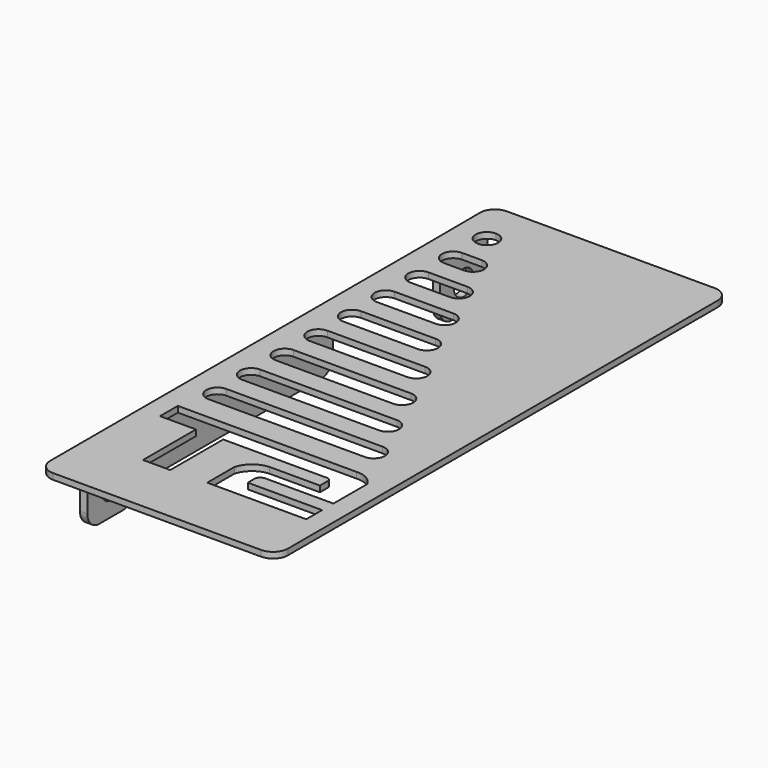
from build123d import *

# Parameters (mm, degrees)
F1_DEPTH = 1.2
F2_DEPTH = 15
F4_D     = 5
F5_R     = 3
F6_DEPTH = 3
F7_DEPTH = 12
F8_R     = 3


# Not quite as in the source:
# - a feature names something its author has since deleted; it is built from what else it names


with BuildPart() as f1:
    # F0 (on Top) → F1 (new body)
    with BuildSketch(Plane.XY):
        Polygon((24, 57.25), (-24, 57.25), (-24.0091441598, 54.25), (-22.5091511277, 54.2454279414), (-22.5091511277, 42.2454279414), (-22.5059426621, 15.2501562063), (-22.5, -34.75), (-22.5, -46.75), (-24, -46.75), (-24, -57.25), (24, -57.25), align=None)
        with BuildLine():
            Line((13.9209458456, -22.2416133583), (-17.6390541544, -22.2416133583))
            ThreePointArc((-17.6390541544, -22.2416133583), (-19.8890541544, -19.9916133583), (-17.6390541544, -17.7416133583))
            Line((-17.6390541544, -17.7416133583), (13.9209458456, -17.7416133583))
            ThreePointArc((13.9209458456, -17.7416133583), (16.1709458456, -19.9916133583), (13.9209458456, -22.2416133583))
        make_face(mode=Mode.SUBTRACT)
        with BuildLine():
            Line((9.9809458456, -13.7416133583), (-17.6390541544, -13.7416133583))
            ThreePointArc((-17.6390541544, -13.7416133583), (-19.8890541544, -11.4916133583), (-17.6390541544, -9.2416133583))
            Line((-17.6390541544, -9.2416133583), (9.9809458456, -9.2416133583))
            ThreePointArc((9.9809458456, -9.2416133583), (12.2309458456, -11.4916133583), (9.9809458456, -13.7416133583))
        make_face(mode=Mode.SUBTRACT)
        with BuildLine():
            Line((6.0409458456, -5.2416133583), (-17.6390541544, -5.2416133583))
            ThreePointArc((-17.6390541544, -5.2416133583), (-19.8890541544, -2.9916133583), (-17.6390541544, -0.7416133583))
            Line((-17.6390541544, -0.7416133583), (6.0409458456, -0.7416133583))
            ThreePointArc((6.0409458456, -0.7416133583), (8.2909458456, -2.9916133583), (6.0409458456, -5.2416133583))
        make_face(mode=Mode.SUBTRACT)
        with BuildLine():
            Line((-19.9999999992, -31.5317022603), (-19.9999999992, -27.0317022603))
            Line((-19.9999999992, -27.0317022603), (16.0951670268, -27.0317022603))
            ThreePointArc((16.0951670268, -27.0317022603), (18.3824934665, -27.555243649), (19.9999999704, -29.25513498))
            Line((19.9999999704, -29.25513498), (19.991580365, -37.75513498))
            Line((19.991580365, -37.75513498), (6.1573753969, -37.7551350426))
            ThreePointArc((6.1573753969, -37.7551350426), (5.4441089744, -38.037790108), (4.9890264818, -38.6554816172))
            Line((4.9890264818, -38.6554816172), (4.9890264818, -40.6197120801))
            Line((4.9890264818, -40.6197120801), (19.9890264818, -40.6197120801))
            Line((19.9890264818, -40.6197120801), (20, -44.6197120801))
            Line((20, -44.6197120801), (0, -44.6197120801))
            Line((0, -44.6197120801), (0, -37.7900532508))
            ThreePointArc((0, -37.7900532508), (1.5958871284, -35.3350022858), (4.3312619815, -34.2900834468))
            Line((4.3312619815, -34.2900834468), (14.5000001306, -34.2900834468))
            Line((14.5000001306, -34.2900834468), (14.5000000048, -32.3122422563))
            ThreePointArc((14.5000000048, -32.3122422563), (14.2713851276, -31.7603171319), (13.7194600008, -31.5317022603))
            Line((13.7194600008, -31.5317022603), (-7.2499999992, -31.5317022603))
            Line((-7.2499999992, -31.5317022603), (-7.2499999992, -44.8960133593))
            Line((-7.2499999992, -44.8960133593), (-12.7499999992, -44.8960133593))
            Line((-12.7499999992, -44.8960133593), (-12.7499999992, -31.5317022603))
            Line((-12.7499999992, -31.5317022603), (-19.9999999992, -31.5317022603))
        make_face(mode=Mode.SUBTRACT)
        with BuildLine():
            Line((2.1009458456, 3.2583866417), (-17.6390541544, 3.2583866417))
            ThreePointArc((-17.6390541544, 3.2583866417), (-19.8890541544, 5.5083866417), (-17.6390541544, 7.7583866417))
            Line((-17.6390541544, 7.7583866417), (2.1009458456, 7.7583866417))
            ThreePointArc((2.1009458456, 7.7583866417), (4.3509458456, 5.5083866417), (2.1009458456, 3.2583866417))
        make_face(mode=Mode.SUBTRACT)
        with BuildLine():
            Line((-2.5590541544, 11.7583866417), (-17.6390541544, 11.7583866417))
            ThreePointArc((-17.6390541544, 11.7583866417), (-19.8890541544, 14.0083866417), (-17.6390541544, 16.2583866417))
            Line((-17.6390541544, 16.2583866417), (-2.5590541544, 16.2583866417))
            ThreePointArc((-2.5590541544, 16.2583866417), (-0.3090541544, 14.0083866417), (-2.5590541544, 11.7583866417))
        make_face(mode=Mode.SUBTRACT)
        with BuildLine():
            Line((-5.7790541544, 20.2583866417), (-17.6390541544, 20.2583866417))
            ThreePointArc((-17.6390541544, 20.2583866417), (-19.8890541544, 22.5083866417), (-17.6390541544, 24.7583866417))
            Line((-17.6390541544, 24.7583866417), (-5.7790541544, 24.7583866417))
            ThreePointArc((-5.7790541544, 24.7583866417), (-3.5290541544, 22.5083866417), (-5.7790541544, 20.2583866417))
        make_face(mode=Mode.SUBTRACT)
        with BuildLine():
            Line((-9.7190541544, 28.7583866417), (-17.6390541544, 28.7583866417))
            ThreePointArc((-17.6390541544, 28.7583866417), (-19.8890541544, 31.0083866417), (-17.6390541544, 33.2583866417))
            Line((-17.6390541544, 33.2583866417), (-9.7190541544, 33.2583866417))
            ThreePointArc((-9.7190541544, 33.2583866417), (-7.4690541544, 31.0083866417), (-9.7190541544, 28.7583866417))
        make_face(mode=Mode.SUBTRACT)
        with BuildLine():
            Line((-13.6590541544, 37.2583866417), (-17.6390541544, 37.2583866417))
            ThreePointArc((-17.6390541544, 37.2583866417), (-19.8890541544, 39.5083866417), (-17.6390541544, 41.7583866417))
            Line((-17.6390541544, 41.7583866417), (-13.6590541544, 41.7583866417))
            ThreePointArc((-13.6590541544, 41.7583866417), (-11.4090541544, 39.5083866417), (-13.6590541544, 37.2583866417))
        make_face(mode=Mode.SUBTRACT)
        with BuildLine():
            Line((-17.5990541544, 45.7583866417), (-17.6390541544, 45.7583866417))
            ThreePointArc((-17.6390541544, 45.7583866417), (-19.8890541544, 48.0083866417), (-17.6390541544, 50.2583866417))
            Line((-17.6390541544, 50.2583866417), (-17.5990541544, 50.2583866417))
            ThreePointArc((-17.5990541544, 50.2583866417), (-15.3490541544, 48.0083866417), (-17.5990541544, 45.7583866417))
        make_face(mode=Mode.SUBTRACT)
    extrude(amount=-F1_DEPTH)

    # F0 (on Top) → F2 (join)
    with BuildSketch(Plane.XY):
        Polygon((-22.5091511277, 54.2454279414), (-24.0091441598, 54.25), (-23.9357289877, 42.2454279414), (-22.5091511277, 42.2454279414), align=None)
        Polygon((-23.997312058, -34.750000301), (-24, -46.75), (-22.5, -46.75), (-22.5, -34.75), align=None)
    extrude(amount=-F2_DEPTH)

    # F4 (through all)
    with Locations(Plane.YZ):
        with Locations((-40.75, -9.5), (48.25, -9.5)):
            Hole(F4_D / 2)

    # F5
    f5_edges = [f1.edges().sort_by_distance(p)[0] for p in [
        (-23.22244, 42.245428, -15),
        (-23.259148, 54.247714, -15),
        (-23.248656, -34.75, -15),
        (-23.25, -46.75, -15),
    ]]
    fillet(f5_edges, radius=F5_R)

    # F0 (on Top) → F6 (join)
    with BuildSketch(Plane.XY):
        Polygon((-22.5091511277, 42.2454279414), (-23.9357289877, 42.2454279414), (-23.9573206897, 15.2499837059), (-22.5059426621, 15.2501562063), align=None)
    extrude(amount=-F6_DEPTH)

    # F0 (on Top) → F7 (join)
    with BuildSketch(Plane.XY):
        Polygon((-22.5059426621, 15.2501562063), (-23.9573206897, 15.2499837059), (-23.997312058, -34.750000301), (-22.5, -34.75), align=None)
    extrude(amount=-F7_DEPTH)

    # F8
    f8_edges = [f1.edges().sort_by_distance(p)[0] for p in [
        (-23.231632, 15.25007, -12),
        (24, 57.25, -0.6),
        (-24, 57.25, -0.6),
        (-24, -57.25, -0.6),
        (24, -57.25, -0.6),
    ]]
    fillet(f8_edges, radius=F8_R)


solid = f1.part
